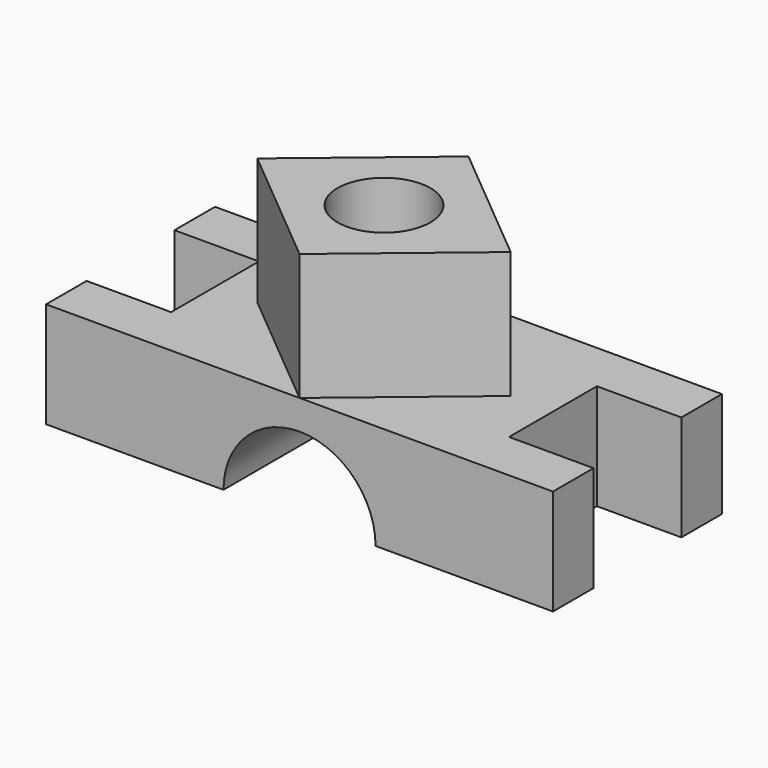
from build123d import *

# Parameters (mm, degrees)
F1_DEPTH = 50
F2_R     = 18
F3_DEPTH = 60
F4_W     = 40
F4_H     = 26
F5_DEPTH = 25
F7_DEPTH = 30
F8_R     = 11
F9_DEPTH = 40


# Not quite as in the source:
# - a feature names something its author has since deleted; it is built from what else it names


with BuildPart() as f1:
    # F0 (on Front) → F1 (new body)
    with BuildSketch(Plane.XZ):
        Polygon((-60, 12.5), (-60, -12.5), (60, -12.5), (60, 12.5), (30, 12.5), (-30, 12.5), align=None)
    extrude(amount=F1_DEPTH)

    # F2 (on face) → F3 (cut)
    with BuildSketch(Plane.XZ.offset(50)):
        with Locations((0, -12.5)):
            Circle(F2_R)
    extrude(amount=-F3_DEPTH, mode=Mode.SUBTRACT)

    # F4 (on face) → F5 (cut)
    with BuildSketch(Plane.XY.offset(12.5)):
        with Locations((-60, -25)):
            Rectangle(F4_W, F4_H)
        with Locations((60, -25)):
            Rectangle(F4_W, F4_H)
    extrude(amount=-F5_DEPTH, mode=Mode.SUBTRACT)

    # F6 (on face) → F7 (join)
    with BuildSketch(Plane.XY.offset(12.5)):
        Polygon((30, -25), (0, 0), (-30, -25), (0, -50), align=None)
    extrude(amount=F7_DEPTH)

    # F8 (on face) → F9 (cut)
    with BuildSketch(Plane.XY.offset(42.5)):
        with Locations((0, -25)):
            Circle(F8_R)
    extrude(amount=-F9_DEPTH, mode=Mode.SUBTRACT)


solid = f1.part
